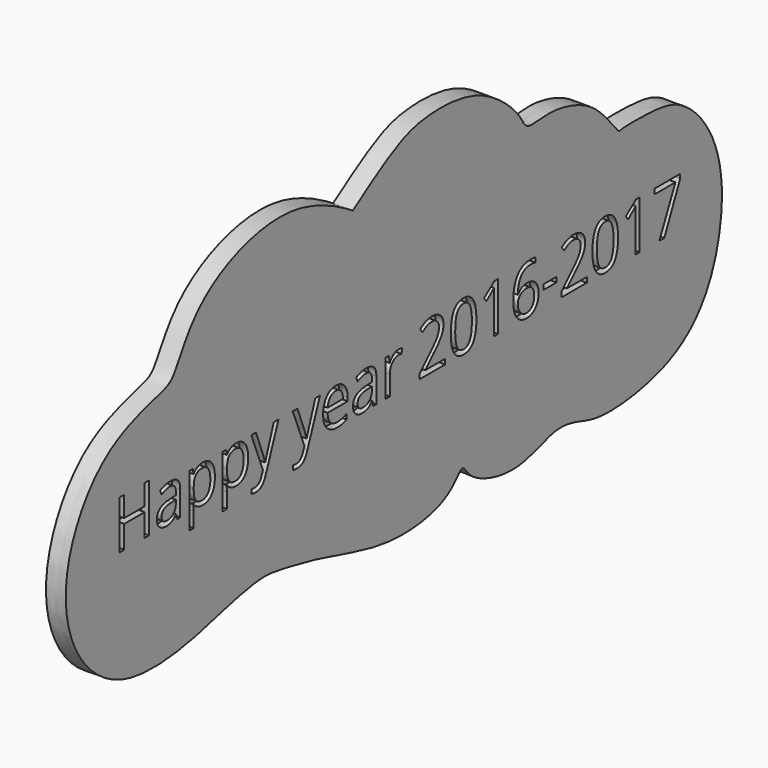
from build123d import *

# Parameters (mm, degrees)
F1_DEPTH     = 3.175
F2_TEXT_SIZE = 10.9043750466
F3_DEPTH     = 1.27


# Not quite as in the source:
# - Text() gives the source's letters only with a copy of the font that has no kerning and outlines rounded to 1/6400 em; it was checked with that copy


with BuildPart() as f1:
    # F0 (on Right) → F1 (new body)
    with BuildSketch(Plane.YZ):
        with BuildLine():
            add(Edge.make_bspline(
                [(-33.7145403028, -20.9618862718), (-36.5021059553, -21.6638208407), (-42.0175526277, -23.2121993293), (-54.5509615349, -23.8846167996), (-64.17831096, -15.5968702881), (-66.5839241775, -2.1027040976), (-58.1790612054, 12.2891428559), (-45.9202368065, 14.7990910653), (-43.1031563737, 16.1413757792), (-39.0999223403, 26.3089337409), (-19.6698477259, 33.2807980028), (-7.5905276932, 25.0606622589), (-7.5340248743, 25.0495120985), (0.8340584072, 30.8552105547), (7.1320080694, 32.6987714076), (18.3562537403, 32.3301360164), (26.2265178644, 25.1870707346), (27.104171483, 22.1483988162), (31.8742979856, 23.177622632), (37.641135872, 21.9063960882), (42.1407677082, 19.3582428638), (45.7921504549, 14.336512078), (46.2971338201, 14.7627899261), (53.2956985189, 14.7777129619), (58.5428841859, 13.7757486868), (64.6047886598, 7.8204935844), (67.6125554575, -2.4004596262), (64.5713100196, -16.1570773415), (55.696222501, -23.4054721668), (42.8376332805, -24.8130815172), (38.4489704421, -23.4051491946), (33.0441333171, -21.7670003254), (25.6371476721, -25.9804326401), (15.8908911444, -22.9731817651), (14.5523086087, -19.4393186339), (12.5143627985, -22.5945544921), (7.62587227, -24.8382319599), (-2.1465593792, -25.0965967235), (-12.5135036544, -21.6686125473), (-21.3553145907, -19.8975700784), (-25.9703970929, -19.1296920561), (-31.0580159354, -20.292949099), (-33.7145403028, -20.9618862718)],
                knots=[0, 0, 0, 0, 0.0270405892, 0.0587075771, 0.089943529, 0.1227282111, 0.1591783018, 0.1902059325, 0.2053815256, 0.2336528391, 0.2751511027, 0.3068649951, 0.3084332639, 0.3359241968, 0.3617229994, 0.3918178927, 0.4209860456, 0.4353005314, 0.4539354308, 0.4763151058, 0.4983056056, 0.5197071872, 0.5255419902, 0.5488772997, 0.571052244, 0.5965663558, 0.6263574919, 0.6598970804, 0.6905449732, 0.7227173442, 0.7424074919, 0.7629274993, 0.7895166264, 0.817883108, 0.8320081007, 0.846549403, 0.8677789358, 0.8962639224, 0.9272857205, 0.954493136, 0.9742305678, 1, 1, 1, 1], degree=3))
        make_face()
    extrude(amount=F1_DEPTH)

    # F2 (on face) → F3 (cut)
    with BuildSketch(Plane.YZ.offset(3.175)):
        with Locations((-55.4277274906, -4.2462100645)):
            Text('Happy year 2016-2017', F2_TEXT_SIZE, font='Open Sans', text_align=(TextAlign.LEFT, TextAlign.BOTTOM))
    extrude(amount=-F3_DEPTH, mode=Mode.SUBTRACT)


solid = f1.part
